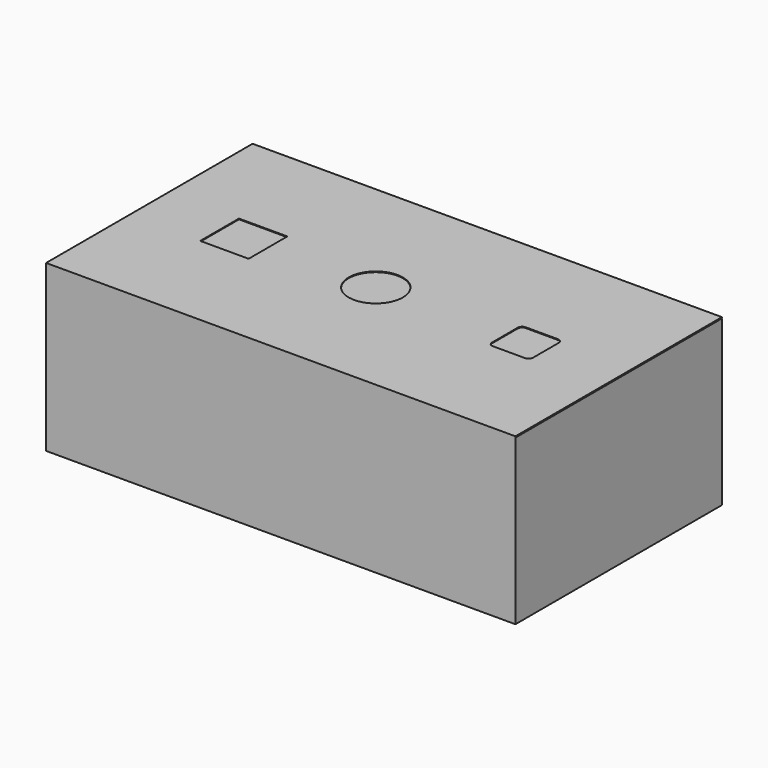
from build123d import *

# Parameters (mm, degrees)
F1_DEPTH = 127
F2_W     = 26.19375
F2_H     = 26.19375
F3_DEPTH = 0.4064


# Not quite as in the source:
# - the dataset's text gives a spline's control points without its knots; the knots are read off the source's solid


with BuildPart() as f1:
    # F0 (on Right) → F1 (new body, symmetric)
    with BuildSketch(Plane.YZ):
        Polygon((-139.7, 0), (0, 0), (0, 88.9), (-139.2936, 88.9), (-139.2936, 89.154), (0, 89.154), (0, 89.5604), (-139.7, 89.5604), align=None)
    extrude(amount=F1_DEPTH, both=True)

    # F2 (on face) → F3 (cut, through all)
    with BuildSketch(Plane.XY.offset(89.5604)):
        with Locations((-75.6309205918, -70.1648127163)):
            Rectangle(F2_W, F2_H)
        with BuildLine():
            add(Edge.make_bspline(
                [(66.3541904082, -59.7497459163), (65.9138814082, -60.1907153163), (65.6568842082, -60.8103483163), (65.6568842082, -61.4337151163)],
                knots=[1, 1, 1, 1, 2, 2, 2, 2], degree=3))
            Line((65.6568842082, -61.4337151163), (65.6568842082, -78.8962151163))
            add(Edge.make_bspline(
                [(65.6568842082, -78.8962151163), (65.6568842082, -79.5194295163), (65.9138814082, -80.1390371163), (66.3541904082, -80.5800065163)],
                knots=[0, 0, 0, 0, 1, 1, 1, 1], degree=3))
            add(Edge.make_bspline(
                [(66.3541904082, -80.5800065163), (66.7951598082, -81.0207981163), (67.4145896082, -81.2774651163), (68.0381342082, -81.2774651163)],
                knots=[1, 1, 1, 1, 2, 2, 2, 2], degree=3))
            Line((68.0381342082, -81.2774651163), (85.5006342082, -81.2774651163))
            add(Edge.make_bspline(
                [(85.5006342082, -81.2774651163), (86.1242042082, -81.2774651163), (86.7436594082, -81.0207981163), (87.1846288082, -80.5800065163)],
                knots=[0, 0, 0, 0, 1, 1, 1, 1], degree=3))
            add(Edge.make_bspline(
                [(87.1846288082, -80.5800065163), (87.6248870082, -80.1390371163), (87.8818842082, -79.5194295163), (87.8818842082, -78.8962151163)],
                knots=[1, 1, 1, 1, 2, 2, 2, 2], degree=3))
            Line((87.8818842082, -78.8962151163), (87.8818842082, -61.4337151163))
            add(Edge.make_bspline(
                [(87.8818842082, -61.4337151163), (87.8818842082, -60.8103483163), (87.6248870082, -60.1907153163), (87.1846288082, -59.7497459163)],
                knots=[0, 0, 0, 0, 1, 1, 1, 1], degree=3))
            add(Edge.make_bspline(
                [(87.1846288082, -59.7497459163), (86.7436594082, -59.3091321163), (86.1242042082, -59.0524651163), (85.5006342082, -59.0524651163)],
                knots=[1, 1, 1, 1, 2, 2, 2, 2], degree=3))
            Line((85.5006342082, -59.0524651163), (68.0381342082, -59.0524651163))
            add(Edge.make_bspline(
                [(68.0381342082, -59.0524651163), (67.4145896082, -59.0524651163), (66.7951598082, -59.3091321163), (66.3541904082, -59.7497459163)],
                knots=[0, 0, 0, 0, 1, 1, 1, 1], degree=3))
        make_face()
        with BuildLine():
            add(Edge.make_bspline(
                [(6.1904042082, -59.7816229163), (3.4722232082, -57.0631117163), (-0.3490797918, -55.4804377163), (-4.1931157918, -55.4804377163)],
                knots=[7, 7, 7, 7, 8, 8, 8, 8], degree=3))
            add(Edge.make_bspline(
                [(-4.1931157918, -55.4804377163), (-8.0371517918, -55.4804377163), (-11.8584547918, -57.0631117163), (-14.5766357918, -59.7816229163)],
                knots=[0, 0, 0, 0, 1, 1, 1, 1], degree=3))
            add(Edge.make_bspline(
                [(-14.5766357918, -59.7816229163), (-17.2951469918, -62.4999817163), (-18.8777955918, -66.3205989163), (-18.8777955918, -70.1649651163), (-18.8777955918, -74.0091789163), (-17.2951469918, -77.8299739163), (-14.5766357918, -80.5484851163)],
                knots=[1, 1, 1, 1, 2, 2, 2, 3, 3, 3, 3], degree=3))
            add(Edge.make_bspline(
                [(-14.5766357918, -80.5484851163), (-11.8584547918, -83.2670217163), (-8.0371517918, -84.8491877163), (-4.1931157918, -84.8491877163), (-0.3490797918, -84.8491877163), (3.4722232082, -83.2670217163), (6.1904042082, -80.5484851163)],
                knots=[3, 3, 3, 3, 4, 4, 4, 5, 5, 5, 5], degree=3))
            add(Edge.make_bspline(
                [(6.1904042082, -80.5484851163), (8.9092964082, -77.8299739163), (10.4912592082, -74.0091789163), (10.4912592082, -70.1649651163), (10.4912592082, -66.3205989163), (8.9092964082, -62.4999817163), (6.1904042082, -59.7816229163)],
                knots=[5, 5, 5, 5, 6, 6, 6, 7, 7, 7, 7], degree=3))
        make_face()
    extrude(amount=-F3_DEPTH, mode=Mode.SUBTRACT)


solid = f1.part
